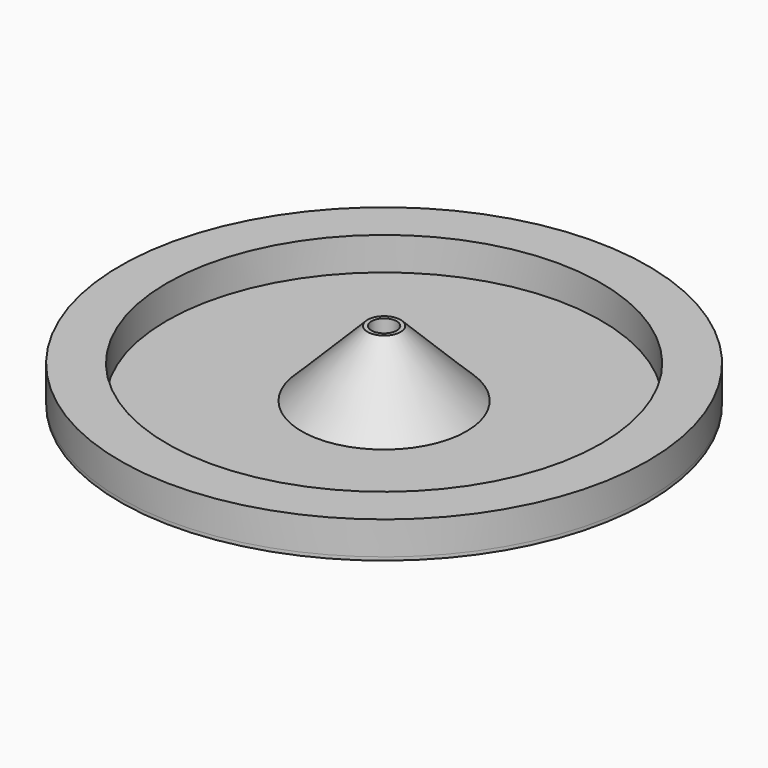
from build123d import *

# Parameters (mm, degrees)
F0_R     = 15
F0_R_2   = 2.3
F1_DEPTH = 12
F0_R_3   = 48
F0_R_4   = 39.5
F2_DEPTH = 0.6
F3_SIZE  = 11.99999
F4_DEPTH = 6


# Not quite as in the source:
# - a fillet or chamfer is up to 0.001 mm smaller than in the source, because OpenCascade refuses the exact size


with BuildPart() as f1:
    # F0 (on Top) → F1 (new body)
    with BuildSketch(Plane.XY):
        Circle(F0_R)
        Circle(F0_R_2, mode=Mode.SUBTRACT)
    extrude(amount=F1_DEPTH)

    # F0 (on Top) → F2 (join)
    with BuildSketch(Plane.XY):
        Circle(F0_R_3)
        Circle(F0_R_4, mode=Mode.SUBTRACT)
        Circle(F0_R_4)
        Circle(F0_R, mode=Mode.SUBTRACT)
        Circle(F0_R)
        Circle(F0_R_2, mode=Mode.SUBTRACT)
    extrude(amount=-F2_DEPTH)

    # F3 (size 12 in the source; OpenCascade refuses exactly that, so slightly less here)
    f3_edges = [f1.edges().sort_by_distance(p)[0] for p in [
        (-15, 0, 12),
    ]]
    chamfer(f3_edges, length=F3_SIZE)

    # F0 (on Top) → F4 (join)
    with BuildSketch(Plane.XY):
        Circle(F0_R_3)
        Circle(F0_R_4, mode=Mode.SUBTRACT)
    extrude(amount=F4_DEPTH)


solid = f1.part
